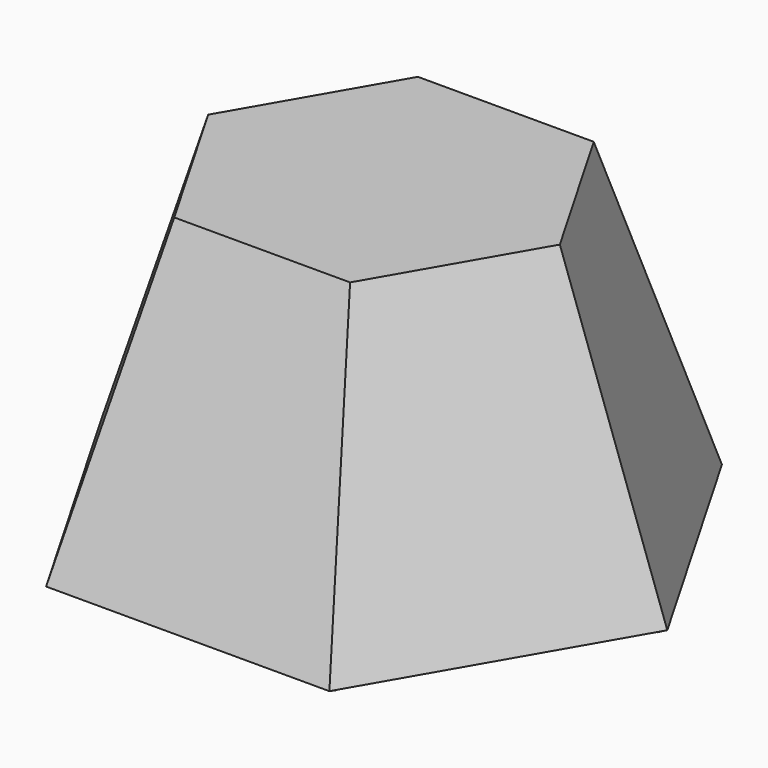
from build123d import *

# Parameters (mm, degrees)
F15_DEPTH = 3.175
F16_DEPTH = 3.175
F17_DEPTH = 3.175
F18_DEPTH = 3.175
F19_DEPTH = 3.175
F20_DEPTH = 3.175
F21_DEPTH = 3.175
F22_W     = 51
F22_H     = 51
F23_DEPTH = 3


with BuildPart() as f15:
    # F14 (on 3pt) → F15 (new body)
    with BuildSketch(Plane(origin=(72.9302177934, -42.1062808751, 25.7316160903), x_dir=(0.4509315595, 0.8782641505, 0.1591000017), z_dir=(0.8282247555, -0.4781757855, 0.2922185356))):
        Polygon((-17.1289231327, 96.8093402992), (-56.8948636851, -17.6873880615), (47.9426159531, -35.3747761231), (47.9426159531, 85.8309615024), align=None)
    extrude(amount=-F15_DEPTH)

    # F4 (on 3pt) → F16 (join)
    with BuildSketch(Plane(origin=(0, -84.2125617502, 25.7316160903), x_dir=(1, 0, 0), z_dir=(0, -0.9563515711, 0.2922185356))):
        Polygon((-32.9955678842, 92.6106952617), (-53.1595260356, -26.9060216653), (53.1595260356, -26.9060216653), (32.9955678842, 92.6106952617), align=None)
    extrude(amount=-F16_DEPTH)

    # F6 (on 3pt) → F17 (join)
    with BuildSketch(Plane(origin=(-72.9302177934, -42.1062808751, 25.7316160903), x_dir=(-0.4509315595, 0.8782641505, 0.1591000017), z_dir=(0.8282247555, 0.4781757855, -0.2922185356))):
        Polygon((-56.8948636851, -17.6873880615), (47.9426159531, -35.3747761231), (47.9426159531, 85.8309615024), (-17.1289231327, 96.8093402992), align=None)
    extrude(amount=F17_DEPTH)

    # F8 (on 3pt) → F18 (join)
    with BuildSketch(Plane(origin=(-72.9302177934, 42.1062808751, 25.7316160903), x_dir=(0.4509315595, 0.8782641505, -0.1591000017), z_dir=(0.8282247555, -0.4781757855, -0.2922185356))):
        Polygon((-47.9426159531, -35.3747761231), (56.8948636851, -17.6873880615), (17.1289231327, 96.8093402992), (-47.9426159531, 85.8309615024), align=None)
    extrude(amount=F18_DEPTH)

    # F10 (on 3pt) → F19 (join)
    with BuildSketch(Plane(origin=(0, 84.2125617502, 25.7316160903), x_dir=(-1, 0, 0), z_dir=(0, 0.9563515711, 0.2922185356))):
        Polygon((-53.1594544198, -26.9060216653), (53.1595260356, -26.9060216653), (32.9955678842, 92.6106952617), (-32.9955678842, 92.6106952617), align=None)
    extrude(amount=-F19_DEPTH)

    # F22 (on face) → F23 (join)
    with BuildSketch(Plane(origin=(0, 84.2125617502, 25.7316160903), x_dir=(-1, 0, 0), z_dir=(0, 0.9563515711, 0.2922185356))):
        with Locations((0, 37.2206158936)):
            Rectangle(F22_W, F22_H)
    extrude(amount=-F23_DEPTH)


with BuildPart() as f20:
    # F12 (on 3pt) → F20 (new body)
    with BuildSketch(Plane(origin=(72.930172863, 42.1063116595, 25.7316002377), x_dir=(-0.4509320281, 0.87826388, -0.159100167), z_dir=(0.8282245004, 0.4781762824, 0.2922184456))):
        Polygon((-47.9426657727, 85.8309615024), (-47.9426657727, -35.3747761231), (56.895113183, -17.6876249146), (17.1287326196, 96.8093622096), align=None)
    extrude(amount=-F20_DEPTH)


with BuildPart() as f21:
    # F2 (on offset) → F21 (new body)
    with BuildSketch(Plane.XY.offset(114.3)):
        Polygon((32.9955678842, 57.15), (-32.9955678842, 57.15), (-65.9911357684, 0), (-32.9955678842, -57.15), (32.9955678842, -57.15), (65.9911357684, 0), align=None)
    extrude(amount=-F21_DEPTH)


solid = Compound([f15.part, f20.part, f21.part])
